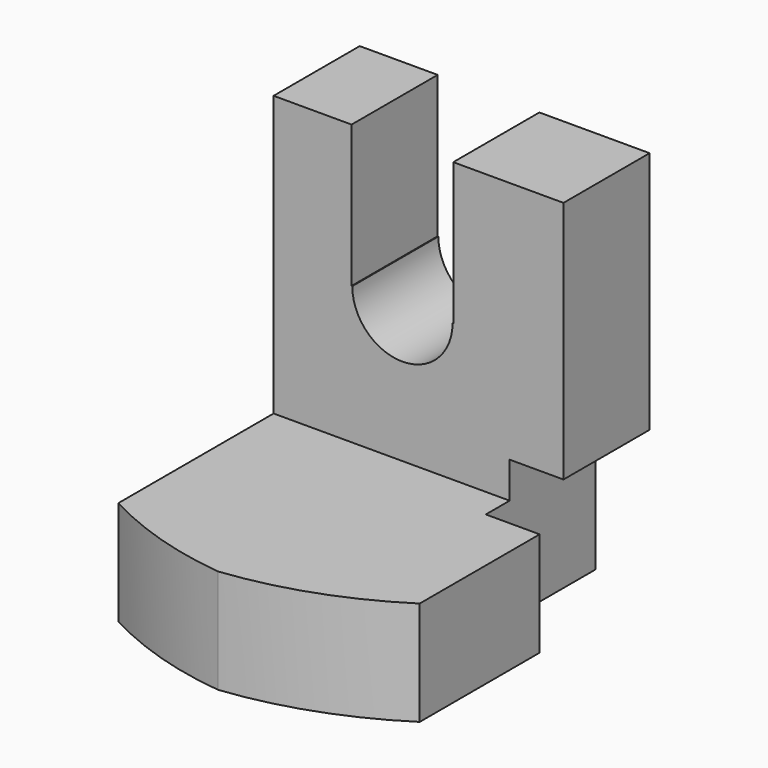
from build123d import *

# Parameters (mm, degrees)
F0_W         = 53.0858039856
F0_H         = 43.5083806515
F1_DEPTH     = 48.3354907483
F2_W         = 29.9567952752
F2_H         = 35.2134015411
F3_DEPTH     = 53.0868039856
F11_W        = 12.8029063344
F11_H        = 17.8795624524
F12_DEPTH    = 13.5525853763
F13_R        = 6.3133849469
F4_DEPTH     = 13.5525853763
F5_SIZE      = 12.7
F14_T1_DEPTH = 107.6402324205
F6_W         = 13.5556794703
F6_H         = 17.6709126681
F15_DEPTH    = 17.3024511896
F7_W         = 6.7778397352
F7_H         = 30.6645780802
F7_W_2       = 9.8140304908
F7_H_2       = 48.3354907483
F8_DEPTH     = 43.2281381166
F9_W         = 6.7778397352
F9_H         = 13.1220892072
F10_DEPTH    = 25.925686927


# Not quite as in the source:
# - a fillet or chamfer that OpenCascade refuses, or shapes differently, is made with other operations: its cross-section is extruded or revolved along the edge and cut away or added


with BuildPart() as f1:
    # F0 (on Top) → F1 (new body)
    with BuildSketch(Plane.XY):
        Rectangle(F0_W, F0_H)
    extrude(amount=F1_DEPTH)

    # F2 (on face) → F3 (cut, through all)
    with BuildSketch(Plane.YZ.offset(26.5429019928)):
        with Locations((-6.7757926881, 30.7287899777)):
            Rectangle(F2_W, F2_H)
    extrude(amount=-F3_DEPTH, mode=Mode.SUBTRACT)

    # F11 (on face) → F12 (cut, through all)
    with BuildSketch(Plane.XZ.offset(-8.2026049495)):
        with Locations((-0.513387844, 39.3957095221)):
            Rectangle(F11_W, F11_H)
    extrude(amount=-F12_DEPTH, mode=Mode.SUBTRACT)

    # F13 (on face) → F4 (cut, through all)
    with BuildSketch(Plane.XZ.offset(-8.2026049495)):
        with Locations((-0.513387844, 30.4559282959)):
            Circle(F13_R)
    extrude(amount=-F4_DEPTH, mode=Mode.SUBTRACT)

    # F5
    f5_edges = [f1.edges().sort_by_distance(p)[0] for p in [
        (26.542902, -21.75419, 6.561045),
        (-26.542902, -21.75419, 6.561045),
    ]]
    chamfer(f5_edges, length=F5_SIZE)

    # F14: fillet of radius 45.6724150938 on 2 edges, made by hand

    # F14_s2 → F14_t1 (cut)
    with BuildSketch(Plane.XY.offset(-47.2590716067)):
        with BuildLine():
            ThreePointArc((5.0607266499, -21.7541903257), (-11.9692421066, -18.4604215607), (-26.5429019928, -9.0541903257))
            Line((-26.5429019928, -9.0541903257), (-13.8429019928, -21.7541903257))
            Line((-13.8429019928, -21.7541903257), (5.0607266499, -21.7541903257))
        make_face()
        with BuildLine():
            ThreePointArc((-5.0607266499, -21.7541903257), (11.9692421066, -18.4604215607), (26.5429019928, -9.0541903257))
            Line((26.5429019928, -9.0541903257), (13.8429019928, -21.7541903257))
            Line((13.8429019928, -21.7541903257), (-5.0607266499, -21.7541903257))
        make_face()
    extrude(amount=F14_T1_DEPTH, mode=Mode.SUBTRACT)

    # F6 (on face) → F15 (cut)
    with BuildSketch(Plane(origin=(0, 21.7541903257, 0), x_dir=(-1, 0, 0), z_dir=(0, 1, 0))):
        with Locations((-19.7650622576, 8.8354563341)):
            Rectangle(F6_W, F6_H)
    extrude(amount=-F15_DEPTH, mode=Mode.SUBTRACT)

    # F7 (on face) → F8 (cut, through all)
    with BuildSketch(Plane(origin=(0, 21.7541903257, 0), x_dir=(-1, 0, 0), z_dir=(0, 1, 0))):
        with Locations((-23.1539821252, 33.0032017082)):
            Rectangle(F7_W, F7_H)
        with Locations((21.6358867474, 24.1677453741)):
            Rectangle(F7_W_2, F7_H_2)
    extrude(amount=-F8_DEPTH, mode=Mode.SUBTRACT)

    # F9 (on face) → F10 (cut, through all)
    with BuildSketch(Plane(origin=(0, 4.4517391361, 0), x_dir=(-1, 0, 0), z_dir=(0, 1, 0))):
        with Locations((-23.1539821252, 6.5610446036)):
            Rectangle(F9_W, F9_H)
    extrude(amount=-F10_DEPTH, mode=Mode.SUBTRACT)


solid = f1.part
